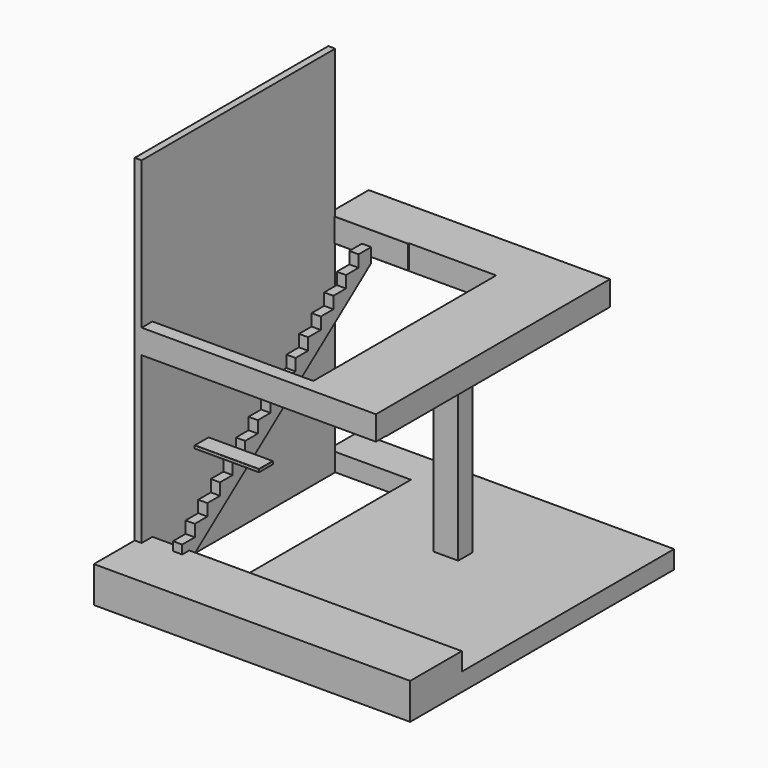
from build123d import *

# Parameters (mm, degrees)
F1_W         = 5229.225
F1_H         = 5454.65
F1_W_2       = 1250.95
F1_H_2       = 3778.25
F2_DEPTH     = 298.45
F4_DEPTH     = 298.45
F6_DEPTH     = 404.8125
F8_DEPTH     = 400.05
F9_W         = 114.3
F9_H         = 4000.5
F10_DEPTH    = 5867.4
F11_W        = 1219.2
F11_H        = 19.05
F12_DEPTH    = 391.16
F15_DEPTH    = 152.4
F16_W        = 407.4945449829
F16_H        = 294.0797805786
F17_DEPTH    = 3027.3625
F20_DEPTH    = 533.4
F21_T1_DEPTH = 311.15


# Not quite as in the source:
# - a fillet or chamfer that OpenCascade refuses, or shapes differently, is made with other operations: its cross-section is extruded or revolved along the edge and cut away or added


with BuildPart() as f2:
    # F1 (on Top) → F2 (new body)
    with BuildSketch(Plane.XY):
        with Locations((2500.3125, 1660.525)):
            Rectangle(F1_W, F1_H)
        with Locations((625.475, 1889.125)):
            Rectangle(F1_W_2, F1_H_2, mode=Mode.SUBTRACT)
    extrude(amount=-F2_DEPTH)

    # F3 (on face) → F4 (join)
    with BuildSketch(Plane.XY):
        Polygon((-114.3, 0), (-114.3, -1066.8), (5114.925, -1066.8), (5114.925, 0), (1250.95, 0), (0, 0), align=None)
    extrude(amount=F4_DEPTH)



with BuildPart() as f6:
    # F5 (on offset) → F6 (new body)
    with BuildSketch(Plane.XY.offset(3432.175)):
        Polygon((0, 0), (0, 3778.25), (2660.65, 3778.25), (2660.65, -1.5875), (3873.5, -1.5875), (3873.5, 4613.6604547501), (3863.975, 4613.6604547501), (-114.3, 4613.6604547501), (-114.3, 0), align=None)
    extrude(amount=-F6_DEPTH)

    # F7 (on face) → F8 (join)
    with BuildSketch(Plane.XY.offset(3432.175)):
        Polygon((0, 0), (-114.3, 0), (-114.3, -222.25), (3873.5, -222.25), (3873.5, -1.5875), (2660.65, -1.5875), (2660.65, 0), align=None)
    extrude(amount=-F8_DEPTH)


with BuildPart() as f2_1:
    add(f2.part)

    add(f6.part)  # F10 merges F6
    # F9 (on face) → F10 (join)
    with BuildSketch(Plane.XY):
        with Locations((-57.15, 1778)):
            Rectangle(F9_W, F9_H)
    extrude(amount=F10_DEPTH)

    # F16 (on face) → F17 (join, through all)
    with BuildSketch(Plane.XY):
        with Locations((2938.0900859833, 2539.3095016479)):
            Rectangle(F16_W, F16_H)
    extrude(amount=F17_DEPTH)


with BuildPart() as f12:
    # F11 (on face) → F12 (new body)
    with BuildSketch(Plane.XY.offset(3432.175)):
        with Locations((609.6, 3768.725)):
            Rectangle(F11_W, F11_H)
    extrude(amount=-F12_DEPTH)


with BuildPart() as f15:
    # F14 (on offset) → F15 (new body)
    with BuildSketch(Plane.YZ.offset(457.2)):
        Polygon((3759.2, 2952.2790994624), (3759.2, 3185.5171875), (3498.85, 3185.5171875), (3498.85, 2989.659375), (3238.5, 2989.659375), (3238.5, 2793.8015625), (2978.15, 2793.8015625), (2978.15, 2597.94375), (2717.8, 2597.94375), (2717.8, 2402.0859375), (2457.45, 2402.0859375), (2457.45, 2206.228125), (2197.1, 2206.228125), (2197.1, 2010.3703125), (1936.75, 2010.3703125), (1936.75, 1814.5125), (1676.4, 1814.5125), (1676.4, 1618.6546875), (1416.05, 1618.6546875), (1416.05, 1422.796875), (1155.7, 1422.796875), (1155.7, 1226.9390625), (895.35, 1226.9390625), (895.35, 1031.08125), (635, 1031.08125), (635, 835.2234375), (374.65, 835.2234375), (374.65, 639.365625), (114.3, 639.365625), (114.3, 443.5078125), (-146.05, 443.5078125), (-146.05, 298.45), (0, 298.45), (0, 124.2833677551), align=None)
    extrude(amount=F15_DEPTH)


with BuildPart() as f20:
    # F19 (on mid) → F20 (new body, symmetric)
    with BuildSketch(Plane.YZ.offset(533.4)):
        with BuildLine():
            Line((876.3, 1226.9390625), (1155.7, 1226.9390625))
            Line((1155.7, 1226.9390625), (1155.7, 1277.7390625))
            Line((1155.7, 1277.7390625), (876.3, 1277.7390625))
            ThreePointArc((876.3, 1277.7390625), (871.8098719395, 1275.8791905605), (869.95, 1271.3890625))
            Line((869.95, 1271.3890625), (869.95, 1233.2890625))
            ThreePointArc((869.95, 1233.2890625), (871.8098719395, 1228.7989344395), (876.3, 1226.9390625))
        make_face()
    extrude(amount=F20_DEPTH, both=True)

    # F21: fillet of radius 6.35 on 4 edges, made by hand

    # F21_s2 → F21_t1 (cut)
    with BuildSketch(Plane.XZ.offset(-1171.575)):
        with BuildLine():
            ThreePointArc((1060.45, 1277.7390625), (1064.9401280605, 1275.8791905605), (1066.8, 1271.3890625))
            Line((1066.8, 1271.3890625), (1066.8, 1277.7390625))
            Line((1066.8, 1277.7390625), (1060.45, 1277.7390625))
        make_face()
        with BuildLine():
            ThreePointArc((1060.45, 1226.9390625), (1064.9401280605, 1228.7989344395), (1066.8, 1233.2890625))
            Line((1066.8, 1233.2890625), (1066.8, 1226.9390625))
            Line((1066.8, 1226.9390625), (1060.45, 1226.9390625))
        make_face()
        with BuildLine():
            ThreePointArc((6.35, 1277.7390625), (1.8598719395, 1275.8791905605), (0, 1271.3890625))
            Line((0, 1271.3890625), (0, 1277.7390625))
            Line((0, 1277.7390625), (6.35, 1277.7390625))
        make_face()
        with BuildLine():
            ThreePointArc((6.35, 1226.9390625), (1.8598719395, 1228.7989344395), (0, 1233.2890625))
            Line((0, 1233.2890625), (0, 1226.9390625))
            Line((0, 1226.9390625), (6.35, 1226.9390625))
        make_face()
    extrude(amount=F21_T1_DEPTH, mode=Mode.SUBTRACT)


solid = Compound([f2_1.part, f12.part, f15.part, f20.part])
